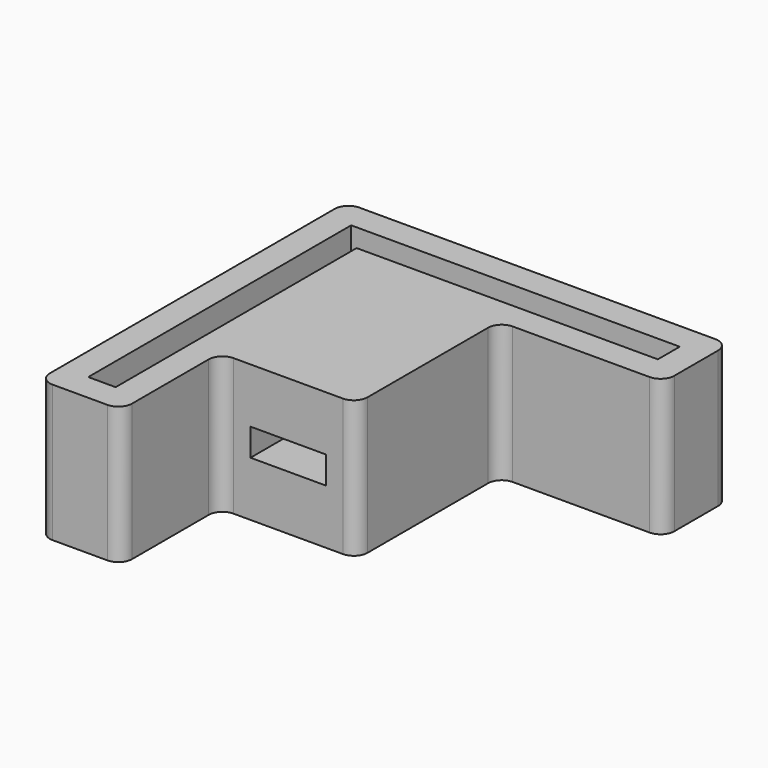
from build123d import *

# Parameters (mm, degrees)
F1_DEPTH    = 5
F2_W        = 10
F2_H        = 10
F3_DEPTH    = 13
F4_R        = 1
F5_W        = 5.5
F5_H        = 2
F7_DEPTH    = 11
F6_W        = 5.5
F6_H        = 2
F8_DEPTH    = 6
F9_T4_DEPTH = 30.5
F9_T7_DEPTH = 5.5


# Not quite as in the source:
# - a fillet or chamfer that OpenCascade refuses, or shapes differently, is made with other operations: its cross-section is extruded or revolved along the edge and cut away or added


with BuildPart() as f1:
    # F0 (on Top) → F1 (new body, symmetric)
    with BuildSketch(Plane.XY):
        Polygon((-6.777402997, 6.5974989831), (15.222597003, 6.5974989831), (15.222597003, 12.5974989831), (-12.777402997, 12.5974989831), (-12.777402997, -15.4025010169), (-6.777402997, -15.4025010169), align=None)
        Polygon((-8.777402997, -13.4025010169), (-10.777402997, -13.4025010169), (-10.777402997, 10.5974989831), (13.222597003, 10.5974989831), (13.222597003, 8.5974989831), (-8.777402997, 8.5974989831), align=None, mode=Mode.SUBTRACT)
    extrude(amount=F1_DEPTH, both=True)

    # F2 (on face) → F3 (join)
    with BuildSketch(Plane.XZ.offset(-6.5974989831)):
        with Locations((-1.777402997, 0)):
            Rectangle(F2_W, F2_H)
    extrude(amount=F3_DEPTH)

    # F4
    f4_edges = [f1.edges().sort_by_distance(p)[0] for p in [
        (3.222597, 6.597499, 0),
        (-12.777403, 12.597499, 0),
        (15.222597, 12.597499, 0),
        (15.222597, 6.597499, 0),
        (-12.777403, -15.402501, 0),
        (-6.777403, -15.402501, 0),
        (3.222597, -6.402501, 0),
        (-6.777403, -6.402501, 0),
    ]]
    fillet(f4_edges, radius=F4_R)

    # F5 (on face) → F7 (cut)
    with BuildSketch(Plane.XZ.offset(6.4025010169)):
        with Locations((-1.777402997, 0)):
            Rectangle(F5_W, F5_H)
    extrude(amount=-F7_DEPTH, mode=Mode.SUBTRACT)

    # F6 (on face) → F8 (cut, through all)
    with BuildSketch(Plane(origin=(0, 0, -5), x_dir=(1, 0, 0), z_dir=(0, 0, -1))):
        with Locations((-1.777402997, -3.5974989831)):
            Rectangle(F6_W, F6_H)
    extrude(amount=-F8_DEPTH, mode=Mode.SUBTRACT)

    # F9: fillet of radius 5 on 2 edges, made by hand


with BuildPart() as f9_tool2:
    # F9_s3 → F9_t4 (new body)
    with BuildSketch(Plane.YZ.offset(13.472597003)):
        with BuildLine():
            ThreePointArc((-0.4025010169, 1), (3.1330328891, -0.4644660941), (4.5974989831, -4))
            Line((4.5974989831, -4), (4.5974989831, 1))
            Line((4.5974989831, 1), (-0.4025010169, 1))
        make_face()
    extrude(amount=-F9_T4_DEPTH)

    split(bisect_by=Plane.YZ.offset(-8.777402997), keep=Keep.TOP)

    split(bisect_by=Plane.YZ.offset(3.222597003), keep=Keep.BOTTOM)


with BuildPart() as f1_1:
    add(f1.part)

    # F9_t1: union F9_tool2
    add(f9_tool2.part)

    # F9_s8 → F9_t7 (cut)
    with BuildSketch(Plane.YZ.offset(-4.527402997)):
        with BuildLine():
            ThreePointArc((2.5974989831, -5), (0.8607971577, -2.1270166538), (-2.3014805024, -1))
            Line((-2.3014805024, -1), (2.5974989831, -1))
            Line((2.5974989831, -1), (2.5974989831, -5))
        make_face()
    extrude(amount=F9_T7_DEPTH, mode=Mode.SUBTRACT)


solid = f1_1.part
